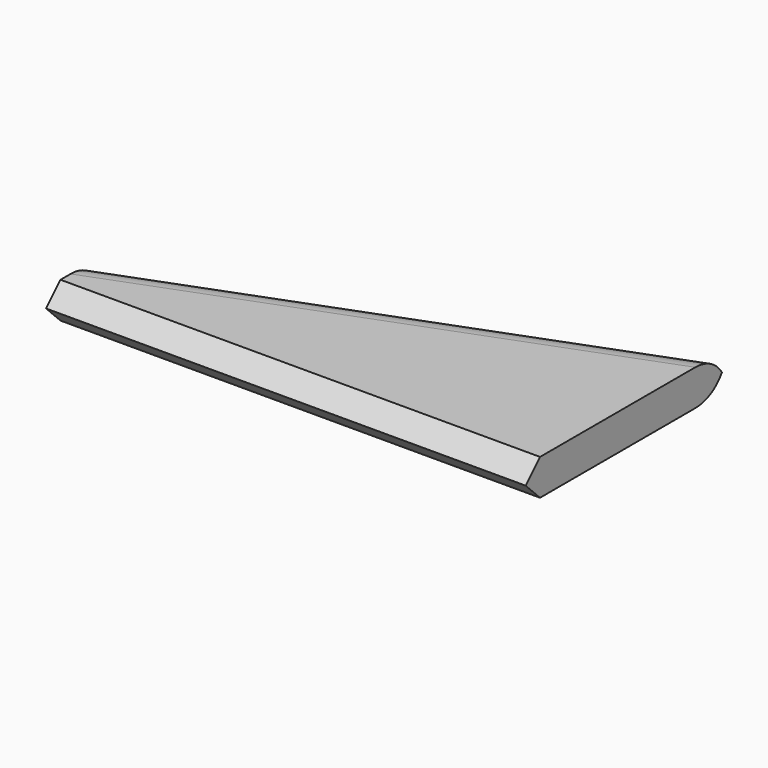
from build123d import *

# Parameters (mm, degrees)
F0_W        = 66.6544139385
F0_H        = 12.0955891907
F1_DEPTH    = 5
F2_T1_DEPTH = 96.2663247468
F3_T1_DEPTH = 92.3712438182


# Not quite as in the source:
# - a fillet or chamfer that OpenCascade refuses, or shapes differently, is made with other operations: its cross-section is extruded or revolved along the edge and cut away or added


with BuildPart() as f1:
    # F0 (on Top) → F1 (new body)
    with BuildSketch(Plane.XY):
        Polygon((-33.3272069693, 6.0477945954), (33.3272069693, 6.0477945954), (33.3272069693, 31.2683843076), align=None)
        Rectangle(F0_W, F0_H)
    extrude(amount=F1_DEPTH)

    # F2: fillet of radius 5 on 2 edges, made by hand

    # F2_s2 → F2_t1 (cut)
    with BuildSketch(Plane(origin=(51.1939340465, 19.37067825, 0), x_dir=(0, 0, 1), z_dir=(-0.9352862544, -0.3538921054, 0))):
        with BuildLine():
            ThreePointArc((0, 17.4506545977), (3.5355339059, 15.9861885036), (5, 12.4506545977))
            Line((5, 12.4506545977), (5, 17.4506545977))
            Line((5, 17.4506545977), (0, 17.4506545977))
        make_face()
        with BuildLine():
            ThreePointArc((5, 17.4506545977), (1.4644660941, 15.9861885036), (0, 12.4506545977))
            Line((0, 12.4506545977), (0, 17.4506545977))
            Line((0, 17.4506545977), (5, 17.4506545977))
        make_face()
    extrude(amount=F2_T1_DEPTH, mode=Mode.SUBTRACT)

    # F3: chamfer of 5 on 2 edges, made by hand

    # F3_s2 → F3_t1 (cut)
    with BuildSketch(Plane.YZ.offset(-46.1856219091)):
        Polygon((-1.0477945954, 5), (-6.0477945954, 0), (-6.0477945954, 5), align=None)
        Polygon((-1.0477945954, 0), (-6.0477945954, 5), (-6.0477945954, 0), align=None)
    extrude(amount=F3_T1_DEPTH, mode=Mode.SUBTRACT)


solid = f1.part
